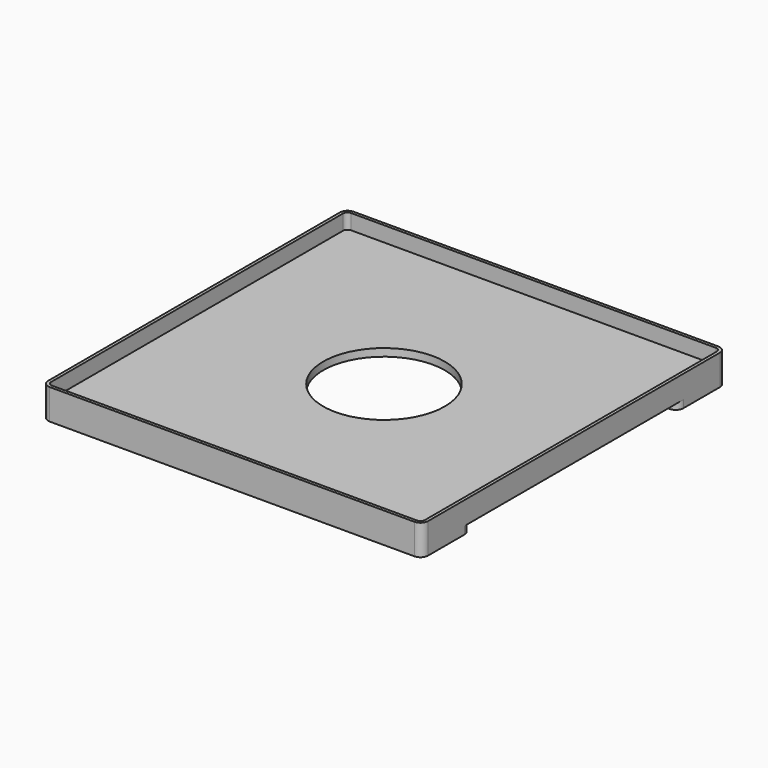
from build123d import *

# Parameters (mm, degrees)
F1_DEPTH = 5
F3_DEPTH = 10
F4_R     = 40
F5_DEPTH = 5.001
F7_DEPTH = 5


# Not quite as in the source:
# - a pattern or mirror of a feature is missing from the dataset's text; its kind, count and spacing are read off the source's solid


with BuildPart() as f1:
    # F0 (on Top) → F1 (new body)
    with BuildSketch(Plane.XY):
        with BuildLine():
            ThreePointArc((125, 120), (123.5355339059, 123.5355339059), (120, 125))
            Line((120, 125), (-120, 125))
            ThreePointArc((-120, 125), (-123.5355339059, 123.5355339059), (-125, 120))
            Line((-125, 120), (-125, -120))
            ThreePointArc((-125, -120), (-123.5355339059, -123.5355339059), (-120, -125))
            Line((-120, -125), (120, -125))
            ThreePointArc((120, -125), (123.5355339059, -123.5355339059), (125, -120))
            Line((125, -120), (125, 120))
        make_face()
    extrude(amount=F1_DEPTH)

    # F2 (on face) → F3 (join)
    with BuildSketch(Plane.XY.offset(5)):
        with BuildLine():
            ThreePointArc((-120, 125), (-123.5355339059, 123.5355339059), (-125, 120))
            Line((-125, 120), (-125, -120))
            ThreePointArc((-125, -120), (-123.5355339059, -123.5355339059), (-120, -125))
            Line((-120, -125), (120, -125))
            ThreePointArc((120, -125), (123.5355339059, -123.5355339059), (125, -120))
            Line((125, -120), (125, 120))
            ThreePointArc((125, 120), (123.5355339059, 123.5355339059), (120, 125))
            Line((120, 125), (-120, 125))
        make_face()
        with BuildLine():
            Line((-120, 123), (120, 123))
            ThreePointArc((120, 123), (122.1213203436, 122.1213203436), (123, 120))
            Line((123, 120), (123, -120))
            ThreePointArc((123, -120), (122.1213203436, -122.1213203436), (120, -123))
            Line((120, -123), (-120, -123))
            ThreePointArc((-120, -123), (-122.1213203436, -122.1213203436), (-123, -120))
            Line((-123, -120), (-123, 120))
            ThreePointArc((-123, 120), (-122.1213203436, 122.1213203436), (-120, 123))
        make_face(mode=Mode.SUBTRACT)
    extrude(amount=F3_DEPTH)

    # F4 (on face) → F5 (cut, through all)
    with BuildSketch(Plane.XY.offset(5)):
        Circle(F4_R)
    extrude(amount=-F5_DEPTH, mode=Mode.SUBTRACT)

    # F6 (on face) → F7 (join)
    with BuildSketch(Plane(origin=(0, 0, 0), x_dir=(1, 0, 0), z_dir=(0, 0, -1))):
        with BuildLine():
            ThreePointArc((-120, 125), (-123.5355339059, 123.5355339059), (-125, 120))
            Line((-125, 120), (-125, 90))
            ThreePointArc((-125, 90), (-123.5355339059, 86.4644660941), (-120, 85))
            Line((-120, 85), (120, 85))
            ThreePointArc((120, 85), (123.5355339059, 86.4644660941), (125, 90))
            Line((125, 90), (125, 120))
            ThreePointArc((125, 120), (123.5355339059, 123.5355339059), (120, 125))
            Line((120, 125), (-120, 125))
        make_face()
        with BuildLine():
            Line((-122, 90), (-122, 120))
            ThreePointArc((-122, 120), (-121.4142135624, 121.4142135624), (-120, 122))
            Line((-120, 122), (120, 122))
            ThreePointArc((120, 122), (121.4142135624, 121.4142135624), (122, 120))
            Line((122, 120), (122, 90))
            ThreePointArc((122, 90), (121.4142135624, 88.5857864376), (120, 88))
            Line((120, 88), (-120, 88))
            ThreePointArc((-120, 88), (-121.4142135624, 88.5857864376), (-122, 90))
        make_face(mode=Mode.SUBTRACT)
    f7 = extrude(amount=F7_DEPTH)

    # F7_copies: F7 across plane
    add(f7.mirror(Plane.ZX))


solid = f1.part
